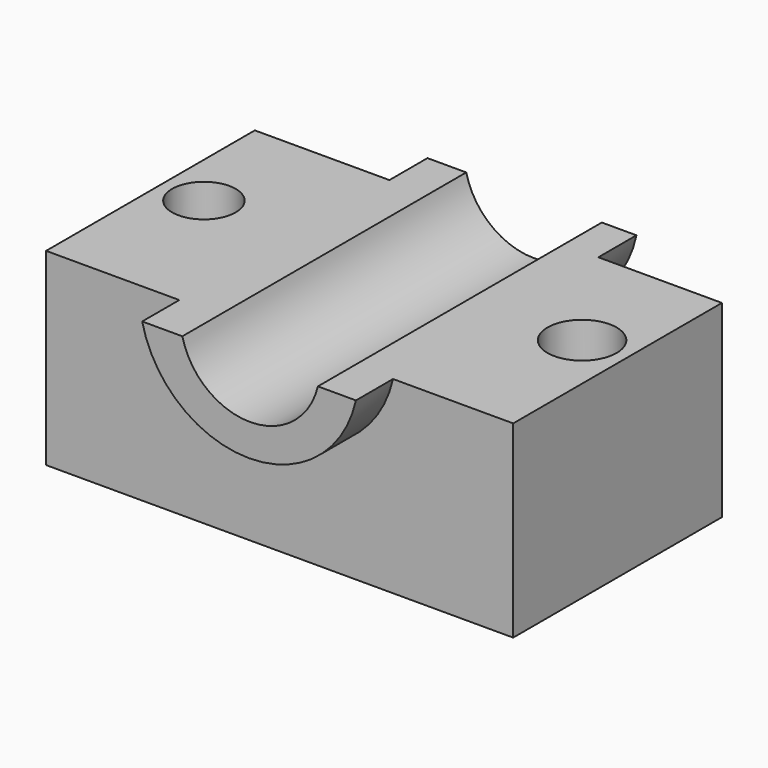
from build123d import *

# Parameters (mm, degrees)
F0_W      = 184.7751736641
F0_H      = 103.2142341137
F1_DEPTH  = 74.6144801378
F3_DEPTH  = 18.3417294174
F5_DEPTH  = 18.8233163208
F7_DEPTH  = 140.3802798519
F8_R      = 12.5990656268
F9_DEPTH  = 74.6154801378
F10_R     = 13.6743893785
F11_DEPTH = 74.6154801378


with BuildPart() as f1:
    # F0 (on Top) → F1 (new body)
    with BuildSketch(Plane.XY):
        with Locations((0, -36.26935184)):
            Rectangle(F0_W, F0_H)
    extrude(amount=F1_DEPTH)

    # F2 (on face) → F3 (join)
    with BuildSketch(Plane.XZ.offset(87.8764688969)):
        with BuildLine():
            Line((44.8529869318, 74.6144801378), (-39.6928861737, 74.6144801378))
            ThreePointArc((-39.6928861737, 74.6144801378), (2.580050379, 40.7354876043), (44.8529869318, 74.6144801378))
        make_face()
    extrude(amount=F3_DEPTH)

    # F4 (on face) → F5 (join)
    with BuildSketch(Plane(origin=(0, 15.3377652168, 0), x_dir=(-1, 0, 0), z_dir=(0, 1, 0))):
        with BuildLine():
            Line((39.1467735171, 74.6144801378), (-43.5126498342, 74.6144801378))
            ThreePointArc((-43.5126498342, 74.6144801378), (-2.1829381585, 41.0193828263), (39.1467735171, 74.6144801378))
        make_face()
    extrude(amount=F5_DEPTH)

    # F6 (on face) → F7 (cut, through all)
    with BuildSketch(Plane.XZ.offset(106.2181983143)):
        with BuildLine():
            Line((29.8108495772, 74.6144801378), (-23.8135512918, 74.6144801378))
            ThreePointArc((-23.8135512918, 74.6144801378), (2.9986491427, 53.4687918706), (29.8108495772, 74.6144801378))
        make_face()
    extrude(amount=-F7_DEPTH, mode=Mode.SUBTRACT)

    # F8 (on face) → F9 (cut, through all)
    with BuildSketch(Plane.XY.offset(74.6144801378)):
        with Locations((-75.3057301044, -31.1868041754)):
            Circle(F8_R)
    extrude(amount=-F9_DEPTH, mode=Mode.SUBTRACT)

    # F10 (on face) → F11 (cut, through all)
    with BuildSketch(Plane.XY.offset(74.6144801378)):
        with Locations((74.2485821247, -31.1318598688)):
            Circle(F10_R)
    extrude(amount=-F11_DEPTH, mode=Mode.SUBTRACT)


solid = f1.part
